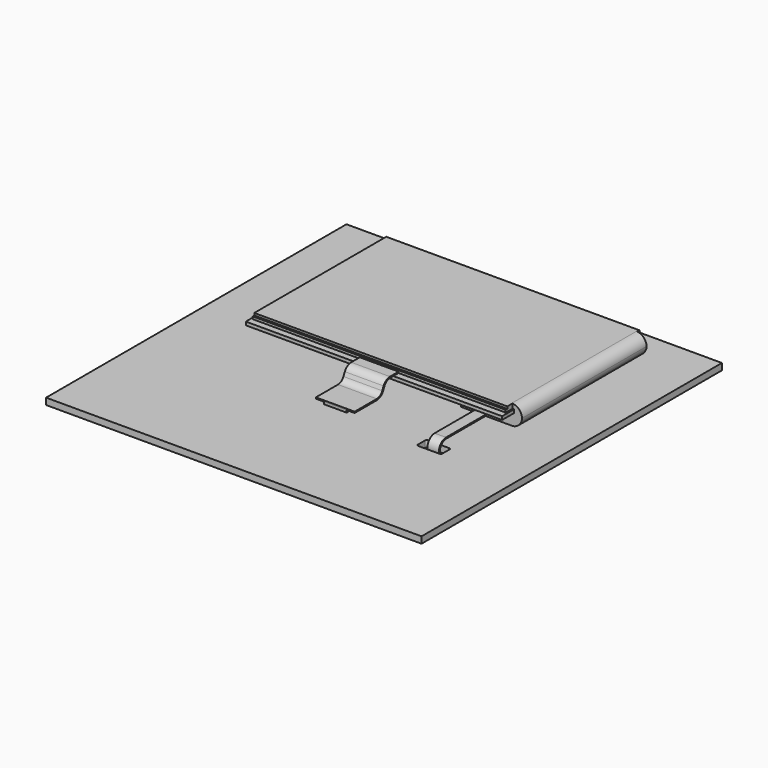
from build123d import *

# Parameters (mm, degrees)
F0_W         = 62.8
F0_H         = 42.82
F1_DEPTH     = 0.81
F2_W         = 15
F2_H         = 38.15
F3_DEPTH     = 2.9
F4_W         = 62
F4_H         = 41.22
F5_DEPTH     = 0.6
F6_W         = 62
F6_H         = 40.42
F7_DEPTH     = 0.54
F8_W         = 2.35
F8_H         = 38.15
F8_W_2       = 62
F9_DEPTH     = 1.95
F10_T1_DEPTH = 50.65
F12_W        = 92
F12_H        = 92
F13_DEPTH    = 1.6
F15_W        = 3
F15_H        = 2.9
F16_DEPTH    = 0.79
F11_W        = 2.8
F11_H        = 0.3
F21_DEPTH    = 1.6
F22_W        = 9.5
F22_H        = 0.3
F26_W        = 5.6
F26_H        = 3.4
F27_DEPTH    = 0.55


# Not quite as in the source:
# - a fillet or chamfer that OpenCascade refuses, or shapes differently, is made with other operations: its cross-section is extruded or revolved along the edge and cut away or added


with BuildPart() as f1:
    # F0 (on Top) → F1 (new body)
    with BuildSketch(Plane.XY):
        Rectangle(F0_W, F0_H)
    extrude(amount=F1_DEPTH)

    # F2 (on face) → F3 (join)
    with BuildSketch(Plane(origin=(0, 0, 0), x_dir=(1, 0, 0), z_dir=(0, 0, -1))):
        with Locations((25.85, -1.335)):
            Rectangle(F2_W, F2_H)
    extrude(amount=F3_DEPTH)

    # F4 (on face) → F5 (join)
    with BuildSketch(Plane.XY.offset(0.81)):
        with Locations((0, 0.8)):
            Rectangle(F4_W, F4_H)
    extrude(amount=F5_DEPTH)

    # F6 (on face) → F7 (join)
    with BuildSketch(Plane.XY.offset(1.41)):
        with Locations((0, 0.9)):
            Rectangle(F6_W, F6_H)
    extrude(amount=F7_DEPTH)

    # F8 (on face) → F9 (join, through all)
    with BuildSketch(Plane.XY.offset(1.95)):
        with Locations((32.175, 1.335)):
            Rectangle(F8_W, F8_H)
        with Locations((0, 1.335)):
            Rectangle(F8_W_2, F8_H)
    extrude(amount=-F9_DEPTH)

    # F10: fillet of radius 2.5 on 2 edges, made by hand

    # F10_s2 → F10_t1 (cut)
    with BuildSketch(Plane.XZ.offset(-26.66)):
        with BuildLine():
            ThreePointArc((30.85, 1.95), (32.617766953, 1.217766953), (33.35, -0.55))
            Line((33.35, -0.55), (33.35, 1.95))
            Line((33.35, 1.95), (30.85, 1.95))
        make_face()
        with BuildLine():
            ThreePointArc((30.85, -2.9), (32.617766953, -2.167766953), (33.35, -0.4))
            Line((33.35, -0.4), (33.35, -2.9))
            Line((33.35, -2.9), (30.85, -2.9))
        make_face()
    extrude(amount=F10_T1_DEPTH, mode=Mode.SUBTRACT)

    # F19: sweep along a path in F18
    with BuildLine(Plane(origin=(24.7, 0, 0), x_dir=(0, -1, 0), z_dir=(-1, 0, 0))) as f19_path:
        Line((17.74, -1.35), (31.94, -1.35))
        ThreePointArc((31.94, -1.35), (33.985, -3.395), (31.94, -5.44))
        Line((31.94, -5.44), (19.3450039609, -5.44))
    # F11 (on face) → F19 (sweep)
    with BuildSketch(Plane.XZ.offset(17.74)):
        with Locations((24.7, -1.35)):
            Rectangle(F11_W, F11_H)
    sweep(path=f19_path.line)

    # F25: sweep along a path in F24
    with BuildLine(Plane.YZ) as f25_path:
        Line((-19.81, 0.96), (-21.41, 0.96))
        Line((-21.41, 0.96), (-22.21, 0.96))
        Line((-22.21, 0.96), (-22.4454795872, 0.96))
        ThreePointArc((-22.4454795872, 0.96), (-23.5142886946, 0.6504576575), (-24.2522561273, -0.1823529082))
        Line((-24.2522561273, -0.1823529082), (-24.6677438727, -1.0576470918))
        ThreePointArc((-24.6677438727, -1.0576470918), (-25.4057113054, -1.8904576575), (-26.4745204128, -2.2))
        Line((-26.4745204128, -2.2), (-26.71, -2.2))
        Line((-26.71, -2.2), (-33.26, -2.2))
    # F22 (on face) → F25 (sweep)
    with BuildSketch(Plane.XZ.offset(19.81)):
        with Locations((0, 0.96)):
            Rectangle(F22_W, F22_H)
    sweep(path=f25_path.line)


with BuildPart() as f13:
    # F12 (on face) → F13 (new body)
    with BuildSketch(Plane(origin=(0, 0, -2.9), x_dir=(1, 0, 0), z_dir=(0, 0, -1))):
        with Locations((0, 18.329)):
            Rectangle(F12_W, F12_H)
    extrude(amount=F13_DEPTH)

    # F15 (on face) → F16 (join)
    with BuildSketch(Plane(origin=(0, 0, -4.5), x_dir=(1, 0, 0), z_dir=(0, 0, -1))):
        with Locations((24.7, 20.7950039609)):
            Rectangle(F15_W, F15_H)
    extrude(amount=F16_DEPTH)

    # F20 (on face) → F21 (cut, through all)
    with BuildSketch(Plane.XY.offset(-2.9)):
        with BuildLine():
            ThreePointArc((27.7, -32.885), (27.5828427125, -32.6021572875), (27.3, -32.485))
            Line((27.3, -32.485), (22.1, -32.485))
            ThreePointArc((22.1, -32.485), (21.8171572875, -32.6021572875), (21.7, -32.885))
            Line((21.7, -32.885), (21.7, -35.085))
            ThreePointArc((21.7, -35.085), (21.8171572875, -35.3678427125), (22.1, -35.485))
            Line((22.1, -35.485), (27.3, -35.485))
            ThreePointArc((27.3, -35.485), (27.5828427125, -35.3678427125), (27.7, -35.085))
            Line((27.7, -35.085), (27.7, -32.885))
        make_face()
    extrude(amount=-F21_DEPTH, mode=Mode.SUBTRACT)

    # F26 (on face) → F27 (join)
    with BuildSketch(Plane.XY.offset(-2.9)):
        with Locations((0, -31.56)):
            Rectangle(F26_W, F26_H)
    extrude(amount=F27_DEPTH)


solid = Compound([f1.part, f13.part])
